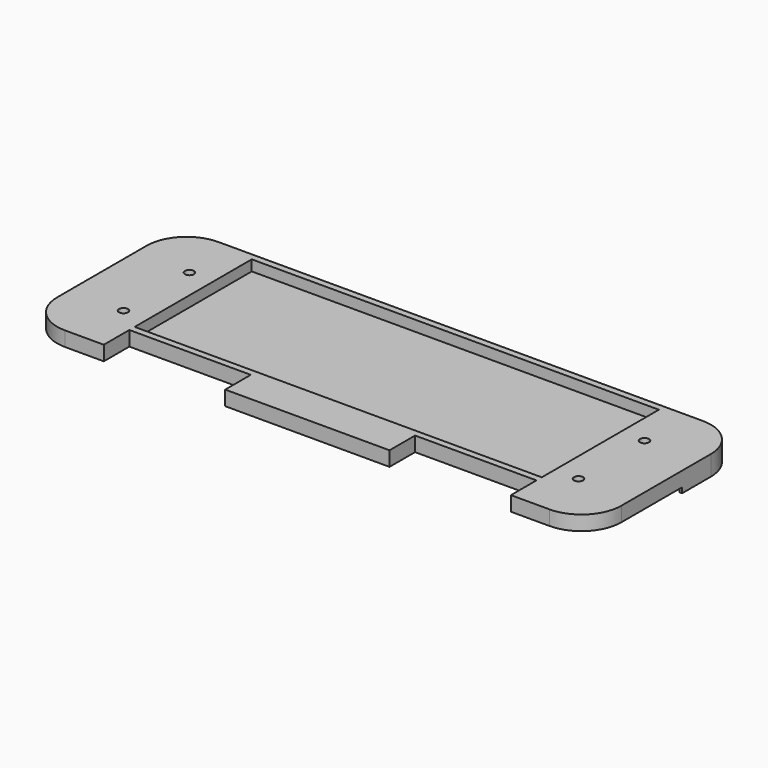
from build123d import *

# Parameters (mm, degrees)
F0_W      = 212
F0_H      = 72
F1_DEPTH  = 5.5
F2_R      = 15
F3_W      = 45.625
F3_H      = 5.5
F4_DEPTH  = 12
F6_DEPTH  = 2
F7_R      = 10.5
F8_R      = 11.5
F9_R      = 14
F10_R     = 15
F11_W     = 153
F11_H     = 55
F12_DEPTH = 4
F14_D     = 3.4


# Not quite as in the source:
# - a feature names something its author has since deleted; it is built from what else it names


with BuildPart() as f1:
    # F0 (on Top) → F1 (new body)
    with BuildSketch(Plane.XY):
        Rectangle(F0_W, F0_H)
    extrude(amount=F1_DEPTH)

    # F2
    f2_edges = [f1.edges().sort_by_distance(p)[0] for p in [
        (-106, -36, 2.75),
        (106, -36, 2.75),
    ]]
    fillet(f2_edges, radius=F2_R)

    # F3 (on face) → F4 (cut)
    with BuildSketch(Plane.XZ.offset(36)):
        with Locations((-53.6875, 2.75)):
            Rectangle(F3_W, F3_H)
        with Locations((53.6875, 2.75)):
            Rectangle(F3_W, F3_H)
    extrude(amount=-F4_DEPTH, mode=Mode.SUBTRACT)

    # F5 (on face) → F6 (join)
    with BuildSketch(Plane(origin=(0, 0, 0), x_dir=(1, 0, 0), z_dir=(0, 0, -1))):
        Polygon((-105, -7.5), (-106, -7.5), (-106, -36), (106, -36), (106, -7.5), (105, -7.5), (105, -35), (-105, -35), align=None)
        Polygon((101.5, -31.5), (-101.5, -31.5), (-101.5, -7.5), (-102.5, -7.5), (-102.5, -32.5), (102.5, -32.5), (102.5, -7.5), (101.5, -7.5), align=None)
    extrude(amount=F6_DEPTH)

    # F7
    f7_edges = [f1.edges().sort_by_distance(p)[0] for p in [
        (101.5, 31.5, -1),
        (-101.5, 31.5, -1),
    ]]
    fillet(f7_edges, radius=F7_R)

    # F8
    f8_edges = [f1.edges().sort_by_distance(p)[0] for p in [
        (102.5, 32.5, -1),
        (-102.5, 32.5, -1),
    ]]
    fillet(f8_edges, radius=F8_R)

    # F9
    f9_edges = [f1.edges().sort_by_distance(p)[0] for p in [
        (105, 35, -1),
        (-105, 35, -1),
    ]]
    fillet(f9_edges, radius=F9_R)

    # F10
    f10_edges = [f1.edges().sort_by_distance(p)[0] for p in [
        (106, 36, 1.75),
        (-106, 36, 1.75),
    ]]
    fillet(f10_edges, radius=F10_R)

    # F11 (on face) → F12 (cut)
    with BuildSketch(Plane.XY.offset(5.5)):
        with Locations((0, 6)):
            Rectangle(F11_W, F11_H)
    extrude(amount=-F12_DEPTH, mode=Mode.SUBTRACT)

    # F14 (through all)
    with Locations(Plane.XY.offset(5.5)):
        with Locations((-85.5, 15.5), (85.5, 15.5), (85.5, -15.5), (-85.5, -15.5)):
            Hole(F14_D / 2)


solid = f1.part
